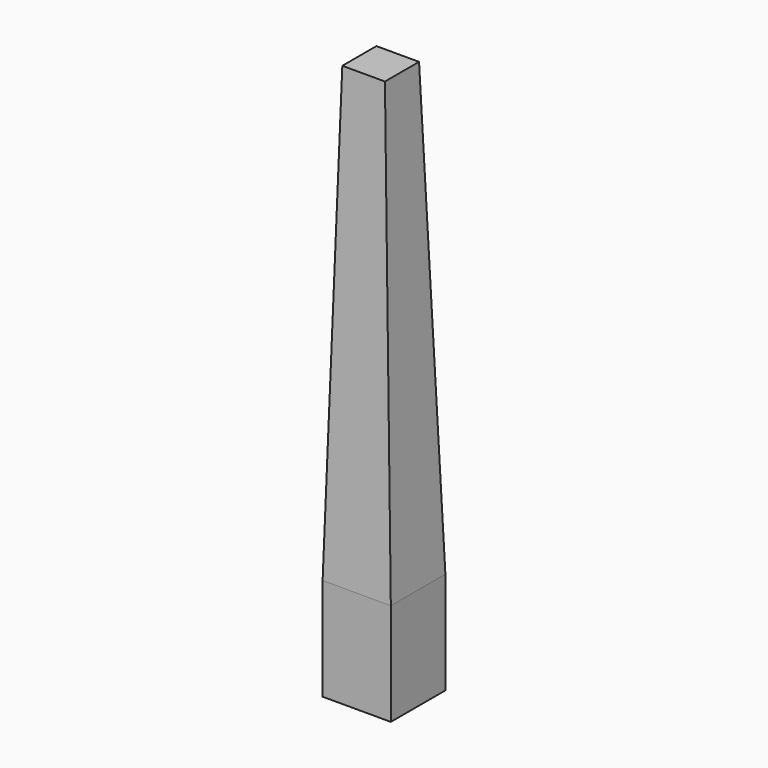
from build123d import *

# Parameters (mm, degrees)
F0_W      = 101.6
F0_H      = 101.6
F1_DEPTH  = 152.4
F1_FACE_W = 101.6
F1_FACE_H = 101.6
F3_W      = 63.5
F3_H      = 63.5


with BuildPart() as f1:
    # F0 (on Top) → F1 (new body)
    with BuildSketch(Plane.XY):
        with Locations((1.8484146567, 0)):
            Rectangle(F0_W, F0_H)
    extrude(amount=F1_DEPTH)

    # F1_face (on face) → F4 section 0
    with BuildSketch(Plane(origin=(1.8484146567, 0, 152.4), x_dir=(1, 0, 0), z_dir=(0, 0, 1))):
        Rectangle(F1_FACE_W, F1_FACE_H)
    # F3 (on offset) → F4 section 1
    with BuildSketch(Plane.XY.offset(812.8)):
        with Locations((-16.7269780412, 17.0467783809)):
            Rectangle(F3_W, F3_H)
    loft()


solid = f1.part
